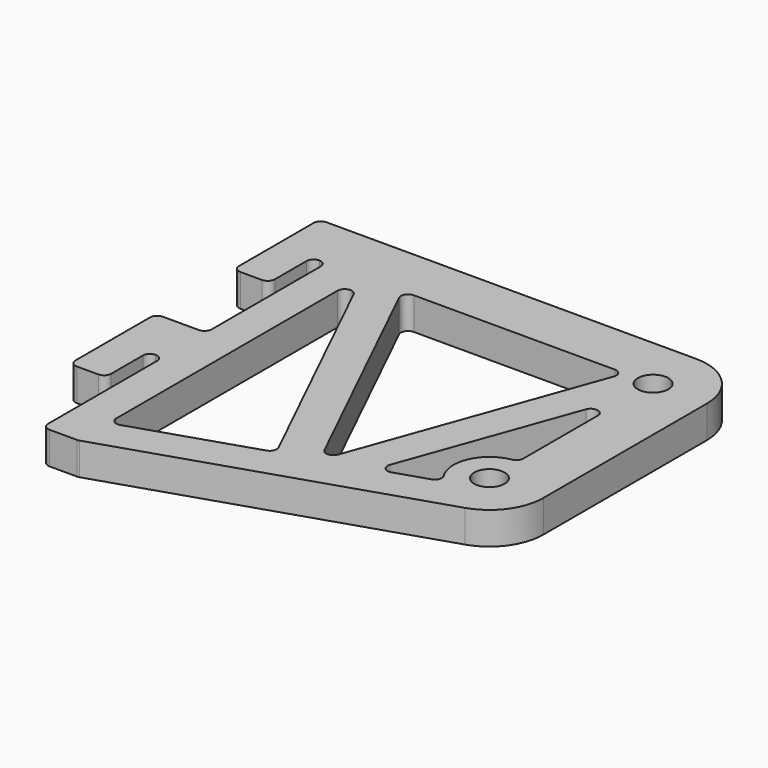
from build123d import *

# Parameters (mm, degrees)
F0_R     = 2.159
F1_DEPTH = 4.572
F2_R     = 1.01599


# Not quite as in the source:
# - a fillet or chamfer is up to 0.001 mm smaller than in the source, because OpenCascade refuses the exact size


with BuildPart() as f1:
    # F0 (on Top) → F1 (new body)
    with BuildSketch(Plane.XY):
        with BuildLine():
            Line((46.228, 28.956), (-7.112, 28.956))
            Line((-7.112, 28.956), (-7.112, 13.716))
            Line((-7.112, 13.716), (-2.032, 13.716))
            Line((-2.032, 13.716), (-2.032, 21.336))
            Line((-2.032, 21.336), (0, 21.336))
            Line((0, 21.336), (0, 0))
            Line((0, 0), (-7.112, 0))
            Line((-7.112, 0), (-7.112, -15.24))
            Line((-7.112, -15.24), (-2.032, -15.24))
            Line((-2.032, -15.24), (-2.032, -7.62))
            Line((-2.032, -7.62), (0, -7.62))
            Line((0, -7.62), (0, -28.956))
            Line((0, -28.956), (5.08, -28.956))
            Line((5.08, -28.956), (48.5757837838, -14.8692972973))
            ThreePointArc((48.5757837838, -14.8692972973), (52.3905689624, -12.1018683363), (53.848, -7.62))
            Line((53.848, -7.62), (53.848, 21.336))
            ThreePointArc((53.848, 21.336), (51.6161536726, 26.7241536726), (46.228, 28.956))
        make_face()
        Polygon((5.08, -23.6162272727), (5.08, 21.336), (23.9526054243, -17.5040766524), align=None, mode=Mode.SUBTRACT)
        with Locations((46.228, -7.62)):
            Circle(F0_R, mode=Mode.SUBTRACT)
        Polygon((28.8326085769, -15.9236210859), (10.7279551462, 21.336), (42.2585858686, 21.336), align=None, mode=Mode.SUBTRACT)
        with BuildLine():
            Line((46.228, 17.3665858686), (46.228, -2.54))
            ThreePointArc((46.228, -2.54), (41.4862817332, -5.7972252255), (42.8252108486, -11.391926032))
            Line((42.8252108486, -11.391926032), (34.9457461194, -13.9437981318))
            Line((34.9457461194, -13.9437981318), (46.228, 17.3665858686))
        make_face(mode=Mode.SUBTRACT)
        with Locations((46.228, 21.336)):
            Circle(F0_R, mode=Mode.SUBTRACT)
    extrude(amount=F1_DEPTH)

    # F2 (radius 1.016 in the source; OpenCascade refuses exactly that, so slightly less here)
    f2_edges = [f1.edges().sort_by_distance(p)[0] for p in [
        (46.228, 17.366586, 2.286),
        (5.08, 21.336, 2.286),
        (10.727955, 21.336, 2.286),
        (42.258586, 21.336, 2.286),
        (23.952605, -17.504077, 2.286),
        (5.08, -23.616227, 2.286),
        (28.832609, -15.923621, 2.286),
        (46.228, -2.54, 2.286),
        (42.825211, -11.391926, 2.286),
        (34.945746, -13.943798, 2.286),
        (5.08, -28.956, 2.286),
        (0, -28.956, 2.286),
        (0, -7.62, 2.286),
        (-2.032, -7.62, 2.286),
        (-2.032, -15.24, 2.286),
        (-7.112, -15.24, 2.286),
        (0, 21.336, 2.286),
        (-2.032, 13.716, 2.286),
        (-7.112, 13.716, 2.286),
        (-7.112, 0, 2.286),
        (0, 0, 2.286),
        (-2.032, 21.336, 2.286),
        (-7.112, 28.956, 2.286),
    ]]
    fillet(f2_edges, radius=F2_R)


solid = f1.part
